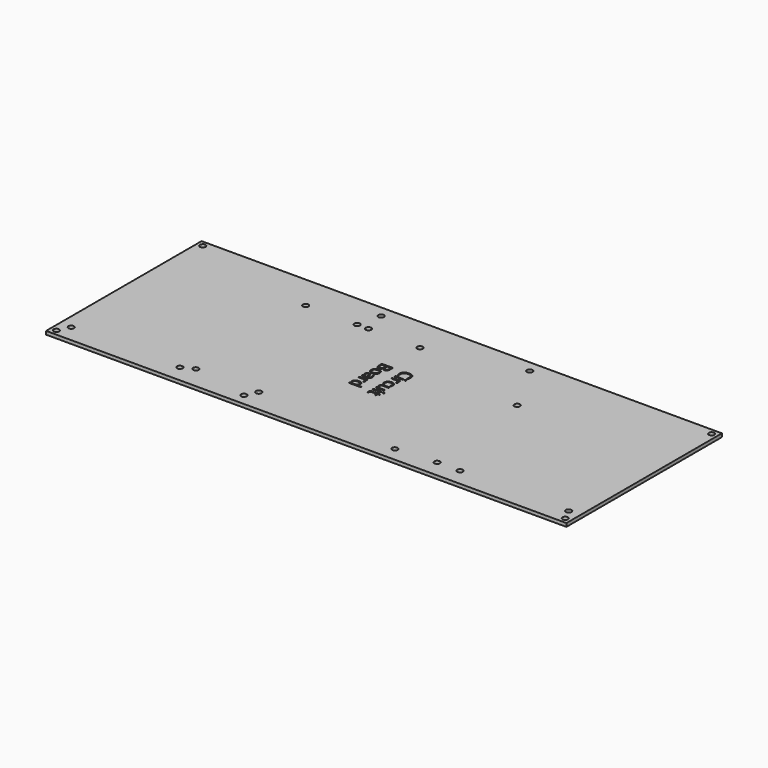
from build123d import *

# Parameters (mm, degrees)
F0_W         = 231.14
F0_H         = 86.36
F0_R         = 1.25
F1_DEPTH     = 1.5
F3_TEXT_SIZE = 6.9444444444
F4_DEPTH     = 1


# Not quite as in the source:
# - Text() gives the source's letters only with a copy of the font that has no kerning and outlines rounded to 1/6400 em; it was checked with that copy


with BuildPart() as f1:
    # F0 (on Top) → F1 (new body)
    with BuildSketch(Plane.XY):
        Rectangle(F0_W, F0_H)
        with Locations((-113.03, -40.64)):
            Circle(F0_R, mode=Mode.SUBTRACT)
        with Locations((-110.49, -35.56)):
            Circle(F0_R, mode=Mode.SUBTRACT)
        with Locations((-62.23, -35.56)):
            Circle(F0_R, mode=Mode.SUBTRACT)
        with Locations((-31.75, -38.1)):
            Circle(F0_R, mode=Mode.SUBTRACT)
        with Locations((-57.15, -33.02)):
            Circle(F0_R, mode=Mode.SUBTRACT)
        with Locations((-29.21, -33.02)):
            Circle(F0_R, mode=Mode.SUBTRACT)
        with Locations((34.29, -36.83)):
            Circle(F0_R, mode=Mode.SUBTRACT)
        with Locations((52.07, -35.56)):
            Circle(F0_R, mode=Mode.SUBTRACT)
        with Locations((62.23, -35.56)):
            Circle(F0_R, mode=Mode.SUBTRACT)
        with Locations((113.03, -40.64)):
            Circle(F0_R, mode=Mode.SUBTRACT)
        with Locations((110.49, -35.56)):
            Circle(F0_R, mode=Mode.SUBTRACT)
        with Locations((-113.03, 40.64)):
            Circle(F0_R, mode=Mode.SUBTRACT)
        with Locations((-57.15, 27.94)):
            Circle(F0_R, mode=Mode.SUBTRACT)
        with Locations((-34.29, 27.94)):
            Circle(F0_R, mode=Mode.SUBTRACT)
        with Locations((-29.21, 27.94)):
            Circle(F0_R, mode=Mode.SUBTRACT)
        with Locations((-6.35, 27.94)):
            Circle(F0_R, mode=Mode.SUBTRACT)
        with Locations((-31.75, 38.1)):
            Circle(F0_R, mode=Mode.SUBTRACT)
        with Locations((46.99, 15.24)):
            Circle(F0_R, mode=Mode.SUBTRACT)
        with Locations((34.29, 38.1)):
            Circle(F0_R, mode=Mode.SUBTRACT)
        with Locations((113.03, 40.64)):
            Circle(F0_R, mode=Mode.SUBTRACT)
    extrude(amount=F1_DEPTH)

    # F3 (on offset) → F4 (cut)
    with BuildSketch(Plane.XY.offset(1.5)):
        with Locations(Location((0.2825735719, 10.9638867262), (0, 0, -90))):
            Text('Circuit', F3_TEXT_SIZE, font='Open Sans', text_align=(TextAlign.LEFT, TextAlign.BOTTOM))
        with Locations(Location((-9.1618708726, 10.9638867262), (0, 0, -90))):
            Text('Board', F3_TEXT_SIZE, font='Open Sans', text_align=(TextAlign.LEFT, TextAlign.BOTTOM))
    extrude(amount=-F4_DEPTH, mode=Mode.SUBTRACT)


solid = f1.part
